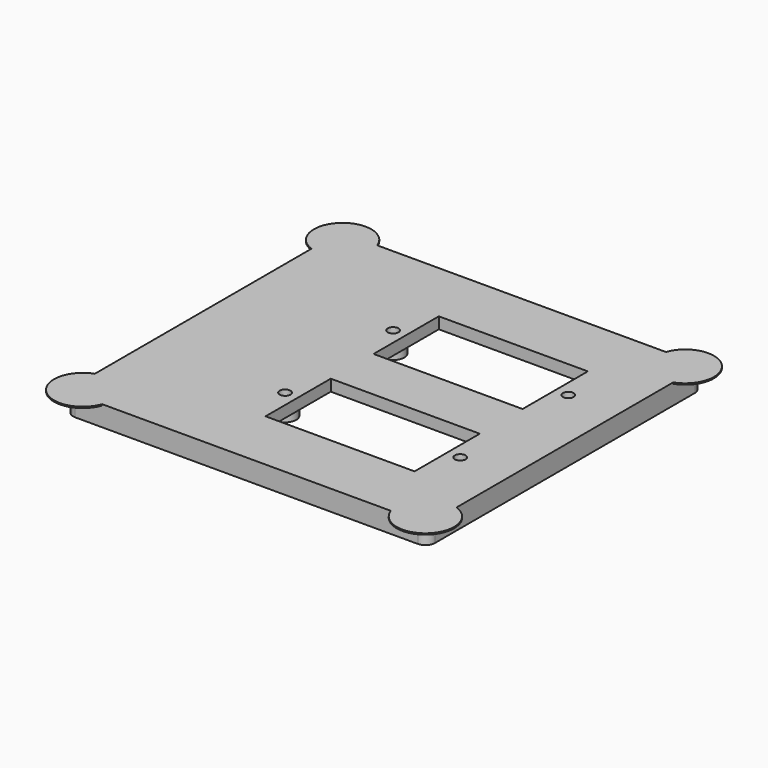
from build123d import *

# Parameters (mm, degrees)
F0_W     = 56.8
F0_H     = 54
F1_DEPTH = 1.8
F2_W     = 23.4
F2_H     = 12.8
F2_R     = 0.85
F3_DEPTH = 1.801
F4_R     = 1.5
F5_R     = 1.75
F5_R_2   = 0.85
F6_DEPTH = 1.4
F7_R     = 4.5
F8_DEPTH = 0.2


# Not quite as in the source:
# - a pattern or mirror of a feature is missing from the dataset's text; its kind, count and spacing are read off the source's solid


with BuildPart() as f1:
    # F0 (on Top) → F1 (new body)
    with BuildSketch(Plane.XY):
        Rectangle(F0_W, F0_H)
    extrude(amount=F1_DEPTH)

    # F2 (on face) → F3 (cut, through all)
    with BuildSketch(Plane.XY.offset(1.8)):
        with Locations((6.7, 10.6)):
            Rectangle(F2_W, F2_H)
        with Locations((-7.05, 10.6)):
            Circle(F2_R)
        with Locations((20.45, 10.6)):
            Circle(F2_R)
    f3 = extrude(amount=-F3_DEPTH, mode=Mode.SUBTRACT)

    # F3_copies: F3 across plane
    add(f3.mirror(Plane(origin=(0, 0, 0), x_dir=(0, 0, -1), z_dir=(0, -1, 0))), mode=Mode.SUBTRACT)

    # F4
    f4_edges = [f1.edges().sort_by_distance(p)[0] for p in [
        (28.4, 27, 0.9),
        (28.4, -27, 0.9),
        (-28.4, -27, 0.9),
        (-28.4, 27, 0.9),
    ]]
    fillet(f4_edges, radius=F4_R)

    # F5 (on face) → F6 (join)
    with BuildSketch(Plane(origin=(0, 0, 0), x_dir=(1, 0, 0), z_dir=(0, 0, -1))):
        with BuildLine():
            Line((-28.4, 25.5), (-28.4, -25.5))
            ThreePointArc((-28.4, -25.5), (-27.9606601718, -26.5606601718), (-26.9, -27))
            Line((-26.9, -27), (26.9, -27))
            ThreePointArc((26.9, -27), (27.9606601718, -26.5606601718), (28.4, -25.5))
            Line((28.4, -25.5), (28.4, 25.5))
            ThreePointArc((28.4, 25.5), (27.9606601718, 26.5606601718), (26.9, 27))
            Line((26.9, 27), (-26.9, 27))
            ThreePointArc((-26.9, 27), (-27.9606601718, 26.5606601718), (-28.4, 25.5))
        make_face()
        with BuildLine():
            Line((26.8, -2), (26.8, -24.4))
            ThreePointArc((26.8, -24.4), (26.5071067812, -25.1071067812), (25.8, -25.4))
            Line((25.8, -25.4), (-25.8, -25.4))
            ThreePointArc((-25.8, -25.4), (-26.5071067812, -25.1071067812), (-26.8, -24.4))
            Line((-26.8, -24.4), (-26.8, -2))
            Line((-26.8, -2), (-26.8, 2))
            Line((-26.8, 2), (-26.8, 24.4))
            ThreePointArc((-26.8, 24.4), (-26.5071067812, 25.1071067812), (-25.8, 25.4))
            Line((-25.8, 25.4), (25.8, 25.4))
            ThreePointArc((25.8, 25.4), (26.5071067812, 25.1071067812), (26.8, 24.4))
            Line((26.8, 24.4), (26.8, 2))
            Line((26.8, 2), (26.8, -2))
        make_face(mode=Mode.SUBTRACT)
        with Locations((-7.05, 10.6)):
            Circle(F5_R)
        with Locations((-7.05, 10.6)):
            Circle(F5_R_2, mode=Mode.SUBTRACT)
        with Locations((-7.05, -10.6)):
            Circle(F5_R)
        with Locations((-7.05, -10.6)):
            Circle(F5_R_2, mode=Mode.SUBTRACT)
        with Locations((20.45, 10.6)):
            Circle(F5_R)
        with Locations((20.45, 10.6)):
            Circle(F5_R_2, mode=Mode.SUBTRACT)
        with Locations((20.45, -10.6)):
            Circle(F5_R)
        with Locations((20.45, -10.6)):
            Circle(F5_R_2, mode=Mode.SUBTRACT)
        with BuildLine():
            ThreePointArc((25.6, -0.8), (26.4485281374, -1.1514718626), (26.8, -2))
            Line((26.8, -2), (26.8, 2))
            ThreePointArc((26.8, 2), (26.4485281374, 1.1514718626), (25.6, 0.8))
            Line((25.6, 0.8), (-25.6, 0.8))
            ThreePointArc((-25.6, 0.8), (-26.4485281374, 1.1514718626), (-26.8, 2))
            Line((-26.8, 2), (-26.8, -2))
            ThreePointArc((-26.8, -2), (-26.4485281374, -1.1514718626), (-25.6, -0.8))
            Line((-25.6, -0.8), (25.6, -0.8))
        make_face()
    extrude(amount=F6_DEPTH)

    # F7 (on face) → F8 (join)
    with BuildSketch(Plane.XY.offset(1.8)):
        with Locations((-26.9, 25.5)):
            Circle(F7_R)
        with Locations((-26.9, -25.5)):
            Circle(F7_R)
        with Locations((26.9, -25.5)):
            Circle(F7_R)
        with Locations((26.9, 25.5)):
            Circle(F7_R)
    extrude(amount=-F8_DEPTH)


solid = f1.part
